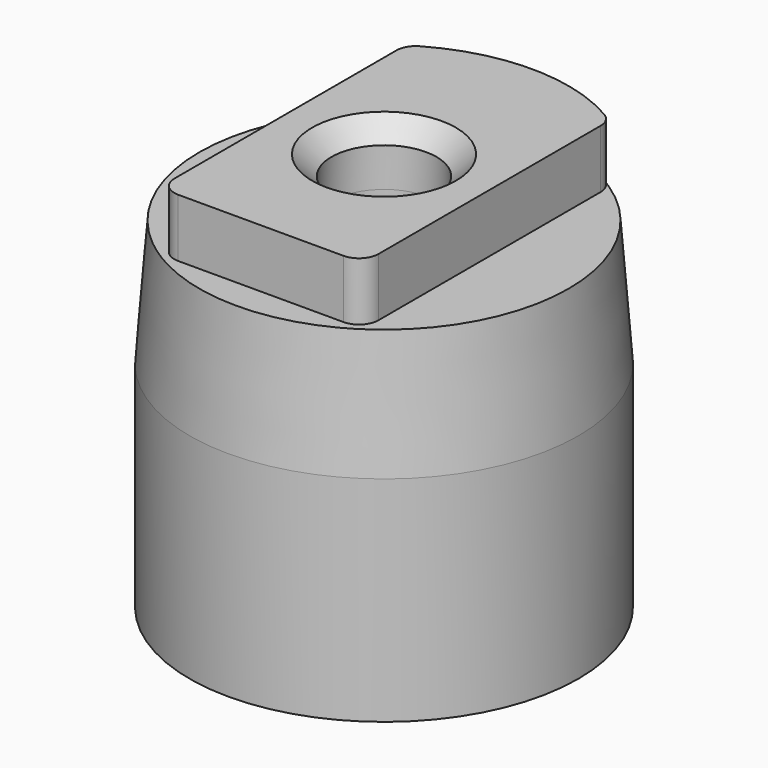
from build123d import *

# Parameters (mm, degrees)
F3_W     = 10.5
F3_H     = 15.8350876221
F3_R     = 2.7
F4_DEPTH = 3
F5_R     = 1
F7_DEPTH = 3
F8_R     = 1
F9_SIZE  = 1


with BuildPart() as f2:
    # F0 (on Front) → F2 (revolve)
    with BuildSketch(Plane.XZ):
        Polygon((4.3, 7), (4.3, 0), (10, 0), (10, 11), (9.5, 17.5), (2.7, 17.5), (2.7, 11.5), align=None)
    revolve(axis=Axis((0, 0, 12.8003526479), (0, 0, -1)))

    # F3 (on face) → F4 (join)
    with BuildSketch(Plane.XY.offset(17.5)):
        Rectangle(F3_W, F3_H)
        Circle(F3_R, mode=Mode.SUBTRACT)
    extrude(amount=F4_DEPTH)

    # F5
    f5_edges = [f2.edges().sort_by_distance(p)[0] for p in [
        (-5.25, -7.917544, 19),
        (5.25, -7.917544, 19),
    ]]
    fillet(f5_edges, radius=F5_R)

    # F6 (on face) → F7 (join)
    with BuildSketch(Plane.XY.offset(17.5)):
        with BuildLine():
            Line((-5.25, 7.9175438111), (5.25, 7.9175438111))
            ThreePointArc((5.25, 7.9175438111), (0, 9.5), (-5.25, 7.9175438111))
        make_face()
    extrude(amount=F7_DEPTH)

    # F8
    f8_edges = [f2.edges().sort_by_distance(p)[0] for p in [
        (5.25, 7.917544, 19),
        (-5.25, 7.917544, 19),
    ]]
    fillet(f8_edges, radius=F8_R)

    # F9
    f9_edges = [f2.edges().sort_by_distance(p)[0] for p in [
        (-2.7, 0, 20.5),
        (2.7, 0, 19),
    ]]
    chamfer(f9_edges, length=F9_SIZE)


solid = f2.part
